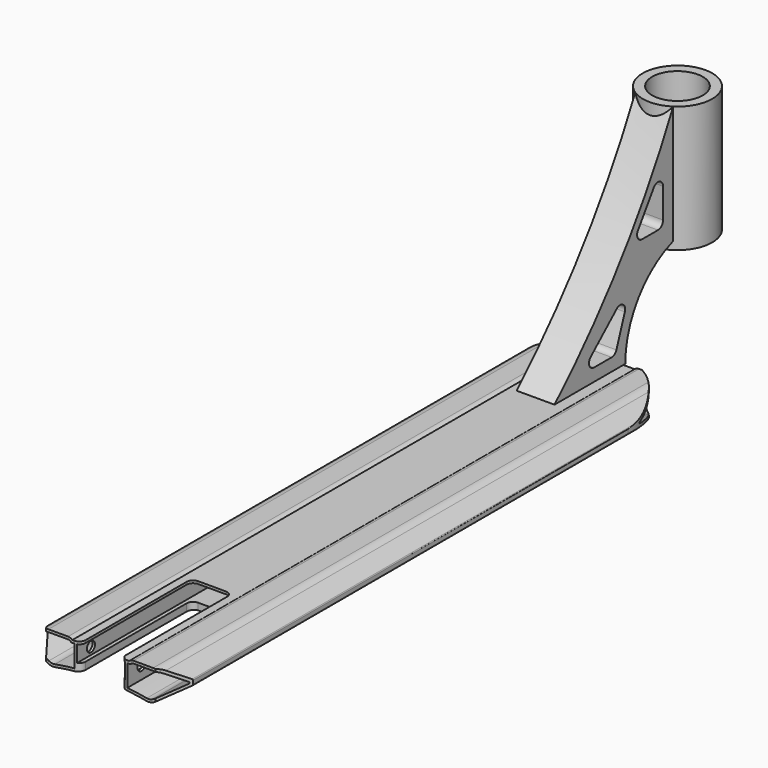
from build123d import *

# Parameters (mm, degrees)
F1_DEPTH       = 250
F2_W           = 38
F2_H           = 13
F3_DEPTH       = 250
F4_T1_DEPTH    = 516.8151717208
F5_R           = 9
F6_R           = 1
F8_DEPTH       = 500.001
F10_DEPTH      = 21.3202008498
F10_DEPTH_BACK = 3.5125286147
F12_DEPTH      = 21.3202009498
F12_DEPTH_BACK = 3.5125287208
F13_F1_R       = 4.9999
F13_F2_R       = 5
F13_F3_R       = 5
F13_F4_R       = 4.9999
F13_F5_R       = 5
F13_F6_R       = 5
F15_DEPTH      = 15
F16_R          = 27.5
F17_DEPTH      = 100
F19_D          = 40
F21_D          = 8
F21_DEPTH      = 45
F21_TIP        = 2.4034424761
F23_DEPTH      = 72.5010001
F24_R          = 5


# Not quite as in the source:
# - a fillet or chamfer that OpenCascade refuses, or shapes differently, is made with other operations: its cross-section is extruded or revolved along the edge and cut away or added
# - a fillet or chamfer is up to 0.001 mm smaller than in the source, because OpenCascade refuses the exact size


with BuildPart() as f1:
    # F0 (on Front) → F1 (new body, symmetric)
    with BuildSketch(Plane.XZ):
        with BuildLine():
            Line((22.5, 20.0192008498), (0, 20.0192008498))
            Line((0, 20.0192008498), (-22.5, 20.0192008498))
            Line((-22.5, 20.0192008498), (-22.5, 21.3192008498))
            Line((-22.5, 21.3192008498), (-44.6950053509, 21.3192008498))
            Line((-44.6950053509, 21.3192008498), (-57.5, 10.5745345625))
            Line((-57.5, 10.5745345625), (-57.5, 6.5745345625))
            Line((-57.5, 6.5745345625), (-39.2176257188, -3.9807991502))
            ThreePointArc((-39.2176257188, -3.9807991502), (0, -0.0980544669), (39.2176257188, -3.9807991502))
            Line((39.2176257188, -3.9807991502), (57.5, 6.5745345625))
            Line((57.5, 6.5745345625), (57.5, 10.5745345625))
            Line((57.5, 10.5745345625), (44.6950053509, 21.3192008498))
            Line((44.6950053509, 21.3192008498), (22.5, 21.3192008498))
            Line((22.5, 21.3192008498), (22.5, 20.0192008498))
        make_face()
    extrude(amount=F1_DEPTH, both=True)

    # F2 (on Front) → F3 (cut, symmetric)
    with BuildSketch(Plane.XZ):
        with Locations((0, 11.5192008498)):
            Rectangle(F2_W, F2_H)
    extrude(amount=F3_DEPTH, both=True, mode=Mode.SUBTRACT)

    # F4: fillet of radius 5 on 2 edges, made by hand

    # F4_s2 → F4_t1 (cut)
    with BuildSketch(Plane.XZ.offset(-258.4075858604)):
        with BuildLine():
            ThreePointArc((25.8630343442, 21.3192008498), (24.0602587064, 20.9828903764), (22.5, 20.0192008498))
            Line((22.5, 20.0192008498), (22.5, 21.3192008498))
            Line((22.5, 21.3192008498), (25.8630343442, 21.3192008498))
        make_face()
        with BuildLine():
            ThreePointArc((-25.8630343442, 21.3192008498), (-24.0602587064, 20.9828903764), (-22.5, 20.0192008498))
            Line((-22.5, 20.0192008498), (-22.5, 21.3192008498))
            Line((-22.5, 21.3192008498), (-25.8630343442, 21.3192008498))
        make_face()
    extrude(amount=F4_T1_DEPTH, mode=Mode.SUBTRACT)

    # F5
    f5_edges = [f1.edges().sort_by_distance(p)[0] for p in [
        (-44.695005, 0, 21.319201),
        (44.695005, 0, 21.319201),
        (-39.217626, 0, -3.980799),
        (39.217626, 0, -3.980799),
    ]]
    fillet(f5_edges, radius=F5_R)

    # F6
    f6_edges = [f1.edges().sort_by_distance(p)[0] for p in [
        (57.5, 0, 6.574535),
        (57.5, 0, 10.574535),
        (-57.5, 0, 10.574535),
        (-57.5, 0, 6.574535),
    ]]
    fillet(f6_edges, radius=F6_R)

    # F7 (on face) → F8 (cut, through all)
    with BuildSketch(Plane.XZ.offset(250)):
        with BuildLine():
            ThreePointArc((25.8630343442, 19.3192008498), (24.4666103398, 18.9743844593), (23.3911929253, 18.0192008498))
            Line((23.3911929253, 18.0192008498), (21, 18.0192008498))
            Line((21, 18.0192008498), (21, 0.807395932))
            ThreePointArc((21, 0.807395932), (28.7006360801, -0.1473768272), (36.3589207949, -1.3972017294))
            ThreePointArc((36.3589207949, -1.3972017294), (38.8121888936, -1.4090660007), (41.1188833968, -0.5737064412))
            Line((41.1188833968, -0.5737064412), (55.5, 7.7292351009))
            ThreePointArc((55.5, 7.7292351009), (56.1089823563, 8.5005501064), (55.7637066814, 9.4206430671))
            Line((55.7637066814, 9.4206430671), (45.9187865103, 17.6815119517))
            ThreePointArc((45.9187865103, 17.6815119517), (43.8134142458, 18.8970491953), (41.4192732425, 19.3192008498))
            Line((41.4192732425, 19.3192008498), (25.8630343442, 19.3192008498))
        make_face()
        with BuildLine():
            ThreePointArc((-36.3589207949, -1.3972017294), (-28.7006360801, -0.1473768272), (-21, 0.807395932))
            Line((-21, 0.807395932), (-21, 18.0192008498))
            Line((-21, 18.0192008498), (-23.3911929253, 18.0192008498))
            ThreePointArc((-23.3911929253, 18.0192008498), (-24.4666103398, 18.9743844593), (-25.8630343442, 19.3192008498))
            Line((-25.8630343442, 19.3192008498), (-41.4192732425, 19.3192008498))
            ThreePointArc((-41.4192732425, 19.3192008498), (-43.8134142458, 18.8970491953), (-45.9187865103, 17.6815119517))
            Line((-45.9187865103, 17.6815119517), (-55.7637066814, 9.4206430671))
            ThreePointArc((-55.7637066814, 9.4206430671), (-56.1089823563, 8.5005501064), (-55.5, 7.7292351009))
            Line((-55.5, 7.7292351009), (-41.1188833968, -0.5737064412))
            ThreePointArc((-41.1188833968, -0.5737064412), (-38.8121888936, -1.4090660007), (-36.3589207949, -1.3972017294))
        make_face()
    extrude(amount=-F8_DEPTH, mode=Mode.SUBTRACT)

    # F9 (on Top) → F10 (cut, two sides)
    with BuildSketch(Plane.XY) as f10_sk:
        with BuildLine():
            ThreePointArc((-57.5, 200), (0.3517310508, 257.4989242097), (57.4956968789, 199.2965510597))
            Line((57.4956968789, 199.2965510597), (58.4830882614, 280))
            Line((58.4830882614, 280), (-57.5, 280))
            Line((-57.5, 280), (-57.5, 200))
        make_face()
    extrude(amount=F10_DEPTH, mode=Mode.SUBTRACT)
    extrude(f10_sk.sketch, amount=-F10_DEPTH_BACK, mode=Mode.SUBTRACT)

    # F11 (on Top) → F12 (cut, two sides)
    with BuildSketch(Plane.XY) as f12_sk:
        Polygon((-43.2975540478, -250), (-68, -216), (-68, -346), (68, -346), (68, -216), (43.2975540478, -250), (16, -250), (16, -140), (-16, -140), (-16, -250), align=None)
    extrude(amount=F12_DEPTH, mode=Mode.SUBTRACT)
    extrude(f12_sk.sketch, amount=-F12_DEPTH_BACK, mode=Mode.SUBTRACT)

    # F13: fillet of radius 5 on 8 edges, made by hand

    # F13_f1 (radius 5 in the source; OpenCascade refuses exactly that, so slightly less here)
    f13_f1_edges = [f1.edges().sort_by_distance(p)[0] for p in [
        (16, -250, 2.1400595465),
    ]]
    fillet(f13_f1_edges, radius=F13_F1_R)

    # F13_f2
    f13_f2_edges = [f1.edges().sort_by_distance(p)[0] for p in [
        (16, -140, 2.1400595465),
    ]]
    fillet(f13_f2_edges, radius=F13_F2_R)

    # F13_f3
    f13_f3_edges = [f1.edges().sort_by_distance(p)[0] for p in [
        (16, -140, 19.0192008498),
    ]]
    fillet(f13_f3_edges, radius=F13_F3_R)

    # F13_f4 (radius 5 in the source; OpenCascade refuses exactly that, so slightly less here)
    f13_f4_edges = [f1.edges().sort_by_distance(p)[0] for p in [
        (-16, -250, 19.0192008498),
    ]]
    fillet(f13_f4_edges, radius=F13_F4_R)

    # F13_f5
    f13_f5_edges = [f1.edges().sort_by_distance(p)[0] for p in [
        (-16, -140, 2.1400595465),
    ]]
    fillet(f13_f5_edges, radius=F13_F5_R)

    # F13_f6
    f13_f6_edges = [f1.edges().sort_by_distance(p)[0] for p in [
        (-16, -140, 19.0192008498),
    ]]
    fillet(f13_f6_edges, radius=F13_F6_R)

    # F21 (one way)
    with BuildSketch(Plane.YZ.offset(21)):
        with Locations((-236, 10.807395932)):
            Circle(F21_D / 2)
    extrude(amount=-F21_DEPTH, mode=Mode.SUBTRACT)
    with Locations(Plane.YZ.offset(21)):
        with Locations((-236, 10.807395932)):
            with Locations((0, 0, -(F21_DEPTH + F21_TIP / 2))):  # 118° drill point
                Cone(0, F21_D / 2, F21_TIP, mode=Mode.SUBTRACT)


with BuildPart() as f15:
    # F14 (on Right) → F15 (new body, symmetric)
    with BuildSketch(Plane.YZ):
        with BuildLine():
            Line((180, 21.3192008498), (250, 21.3192008498))
            ThreePointArc((250, 21.3192008498), (263.064685674, 62.04228991), (297.3819995028, 87.5643973059))
            Line((297.3819995028, 87.5643973059), (297.3819995028, 81.3192008498))
            Line((297.3819995028, 81.3192008498), (343.3819995028, 81.3192008498))
            Line((343.3819995028, 81.3192008498), (343.3819995028, 181.3192008498))
            Line((343.3819995028, 181.3192008498), (297.3819995028, 181.3192008498))
            ThreePointArc((297.3819995028, 181.3192008498), (245.9666940414, 95.9814787028), (180, 21.3192008498))
        make_face()
    extrude(amount=F15_DEPTH, both=True)

    # F16 (on face) → F17 (join, through all)
    with BuildSketch(Plane.XY.offset(181.3192008498)):
        with Locations((0, 320.3819995028)):
            Circle(F16_R)
    extrude(amount=-F17_DEPTH)

    # F19 (through all)
    with Locations(Plane.XY.offset(181.3192008498)):
        with Locations((0, 320.3819995028)):
            Hole(F19_D / 2)

    # F22 (on face) → F23 (cut, through all)
    with BuildSketch(Plane.YZ.offset(15)):
        Polygon((287.3331383596, 146.3192008499), (257.3331383596, 101.3192008499), (287.3331383596, 101.3192008499), align=None)
        Polygon((256.378660542, 76.3192008498), (206, 31.3192008498), (240, 31.3192008498), align=None)
    extrude(amount=-F23_DEPTH, mode=Mode.SUBTRACT)

    # F24
    f24_edges = [f15.edges().sort_by_distance(p)[0] for p in [
        (0, 287.333138, 146.319201),
        (0, 257.333138, 101.319201),
        (0, 287.333138, 101.319201),
        (0, 240, 31.319201),
        (0, 256.378661, 76.319201),
        (0, 206, 31.319201),
    ]]
    fillet(f24_edges, radius=F24_R)


solid = Compound([f1.part, f15.part])
